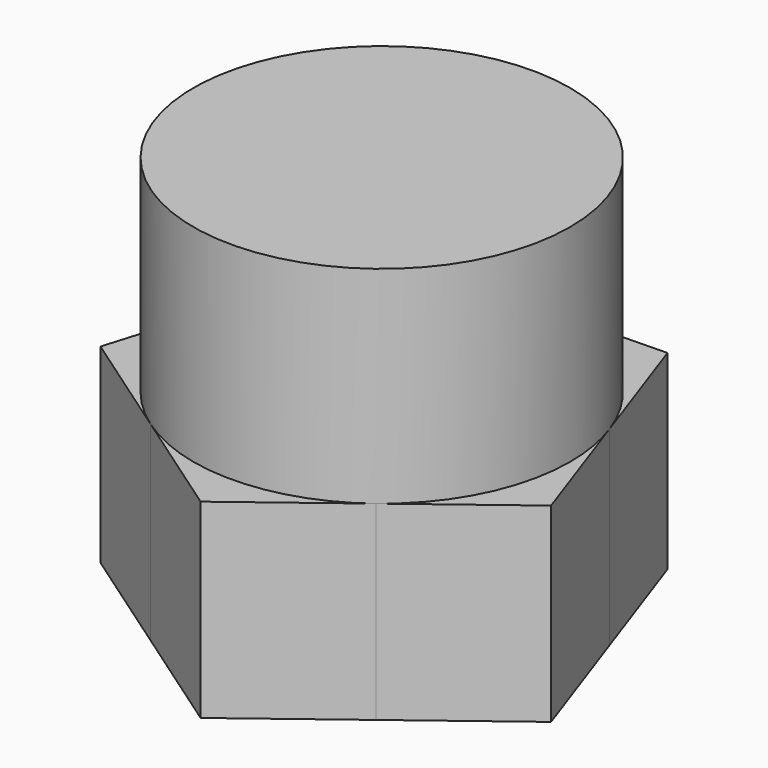
from build123d import *

# Parameters (mm, degrees)
F0_R     = 50
F1_DEPTH = 54.864
F3_DEPTH = 50.546


with BuildPart() as f1:
    # F0 (on Top) → F1 (new body)
    with BuildSketch(Plane.XY):
        Circle(F0_R)
    extrude(amount=F1_DEPTH)

    # F2 (on face) → F3 (join)
    with BuildSketch(Plane(origin=(0, 0, 0), x_dir=(1, 0, 0), z_dir=(0, 0, -1))):
        with BuildLine():
            Line((30.2700951576, 39.7959965216), (1.3566113452, 61.7885079781))
            Line((1.3566113452, 61.7885079781), (-28.494267061, 41.0862111256))
            ThreePointArc((-28.494267061, 41.0862111256), (1.0975221129, 49.9879530008), (30.2700951576, 39.7959965216))
        make_face()
        with BuildLine():
            Line((59.1835791051, 17.8034849624), (30.2700951576, 39.7959965216))
            ThreePointArc((30.2700951576, 39.7959965216), (44.7967898285, 22.209178757), (50, 0))
            ThreePointArc((50, 0), (49.2955920393, -8.3632891551), (47.2022157803, -16.4909316118))
            Line((47.2022157803, -16.4909316118), (59.1835791051, 17.8034849624))
        make_face()
        with BuildLine():
            ThreePointArc((50, 0), (44.7967898285, 22.209178757), (30.2700951576, 39.7959965216))
            ThreePointArc((30.2700951576, 39.7959965216), (1.0975221129, 49.9879530008), (-28.494267061, 41.0862111256))
            ThreePointArc((-28.494267061, 41.0862111256), (-47.2022150962, 16.49093357), (-47.8805218829, -14.4033199027))
            ThreePointArc((-47.8805218829, -14.4033199027), (-30.2700960741, -39.7959958245), (-1.097521687, -49.9879530102))
            ThreePointArc((-1.097521687, -49.9879530102), (28.4942681078, -41.0862103996), (47.2022157803, -16.4909316118))
            ThreePointArc((47.2022157803, -16.4909316118), (49.2955920393, -8.3632891551), (50, 0))
        make_face()
        with BuildLine():
            ThreePointArc((-47.8805218829, -14.4033199027), (-47.2022150962, 16.49093357), (-28.494267061, 41.0862111256))
            Line((-28.494267061, 41.0862111256), (-58.3451471843, 20.3839130822))
            Line((-58.3451471843, 20.3839130822), (-47.8805218829, -14.4033199027))
        make_face()
        with BuildLine():
            ThreePointArc((-1.097521687, -49.9879530102), (-30.2700960741, -39.7959958245), (-47.8805218829, -14.4033199027))
            Line((-47.8805218829, -14.4033199027), (-37.4158953837, -49.1905568696))
            Line((-37.4158953837, -49.1905568696), (-1.097521687, -49.9879530102))
        make_face()
        with BuildLine():
            Line((35.2208521177, -50.7853491531), (47.2022157803, -16.4909316118))
            ThreePointArc((47.2022157803, -16.4909316118), (28.4942681078, -41.0862103996), (-1.097521687, -49.9879530102))
            Line((-1.097521687, -49.9879530102), (35.2208521177, -50.7853491531))
        make_face()
    extrude(amount=F3_DEPTH)


solid = f1.part
